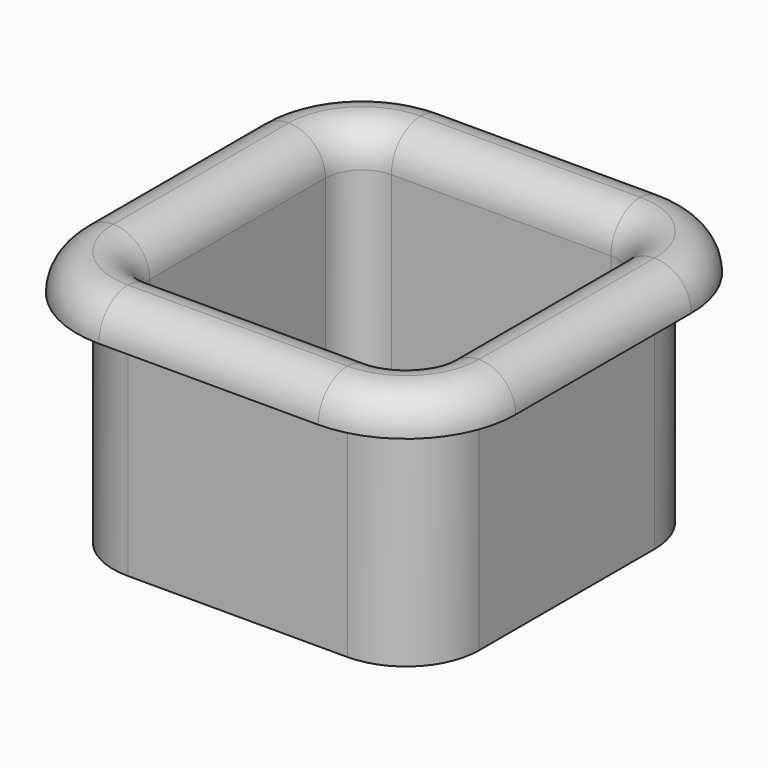
from build123d import *

# Parameters (mm, degrees)
F1_DEPTH = 6.35
F2_DEPTH = 38.1
F3_R     = 6.34999


# Not quite as in the source:
# - a fillet or chamfer is up to 0.001 mm smaller than in the source, because OpenCascade refuses the exact size


with BuildPart() as f1:
    # F0 (on Top) → F1 (new body)
    with BuildSketch(Plane.XY):
        with BuildLine():
            Line((-19.05, -38.1000031829), (19.05, -38.1000031829))
            ThreePointArc((19.05, -38.1000031829), (32.5203864322, -32.5203864322), (38.1000031829, -19.05))
            Line((38.1000031829, -19.05), (38.1000031829, 19.05))
            ThreePointArc((38.1000031829, 19.05), (32.5203864322, 32.5203864322), (19.05, 38.1000031829))
            Line((19.05, 38.1000031829), (-19.05, 38.1000031829))
            ThreePointArc((-19.05, 38.1000031829), (-32.5203864322, 32.5203864322), (-38.1000031829, 19.05))
            Line((-38.1000031829, 19.05), (-38.1000031829, -19.05))
            ThreePointArc((-38.1000031829, -19.05), (-32.5203864322, -32.5203864322), (-19.05, -38.1000031829))
        make_face()
        with BuildLine():
            ThreePointArc((-19.05, -31.75), (-28.0302561211, -28.0302561211), (-31.75, -19.05))
            Line((-31.75, -19.05), (-31.75, 19.05))
            ThreePointArc((-31.75, 19.05), (-28.0302561211, 28.0302561211), (-19.05, 31.75))
            Line((-19.05, 31.75), (19.05, 31.75))
            ThreePointArc((19.05, 31.75), (28.0302561211, 28.0302561211), (31.75, 19.05))
            Line((31.75, 19.05), (31.75, -19.05))
            ThreePointArc((31.75, -19.05), (28.0302561211, -28.0302561211), (19.05, -31.75))
            Line((19.05, -31.75), (-19.05, -31.75))
        make_face(mode=Mode.SUBTRACT)
        with BuildLine():
            Line((-31.75, 19.05), (-31.75, -19.05))
            ThreePointArc((-31.75, -19.05), (-28.0302561211, -28.0302561211), (-19.05, -31.75))
            Line((-19.05, -31.75), (19.05, -31.75))
            ThreePointArc((19.05, -31.75), (28.0302561211, -28.0302561211), (31.75, -19.05))
            Line((31.75, -19.05), (31.75, 19.05))
            ThreePointArc((31.75, 19.05), (28.0302561211, 28.0302561211), (19.05, 31.75))
            Line((19.05, 31.75), (-19.05, 31.75))
            ThreePointArc((-19.05, 31.75), (-28.0302561211, 28.0302561211), (-31.75, 19.05))
        make_face()
        with BuildLine():
            Line((19.05, -25.4), (-19.05, -25.4))
            ThreePointArc((-19.05, -25.4), (-23.5401280605, -23.5401280605), (-25.4, -19.05))
            Line((-25.4, -19.05), (-25.4, 19.05))
            ThreePointArc((-25.4, 19.05), (-23.5401280605, 23.5401280605), (-19.05, 25.4))
            Line((-19.05, 25.4), (19.05, 25.4))
            ThreePointArc((19.05, 25.4), (23.5401280605, 23.5401280605), (25.4, 19.05))
            Line((25.4, 19.05), (25.4, -19.05))
            ThreePointArc((25.4, -19.05), (23.5401280605, -23.5401280605), (19.05, -25.4))
        make_face(mode=Mode.SUBTRACT)
    extrude(amount=F1_DEPTH)

    # F0 (on Top) → F2 (join)
    with BuildSketch(Plane.XY):
        with BuildLine():
            Line((-31.75, 19.05), (-31.75, -19.05))
            ThreePointArc((-31.75, -19.05), (-28.0302561211, -28.0302561211), (-19.05, -31.75))
            Line((-19.05, -31.75), (19.05, -31.75))
            ThreePointArc((19.05, -31.75), (28.0302561211, -28.0302561211), (31.75, -19.05))
            Line((31.75, -19.05), (31.75, 19.05))
            ThreePointArc((31.75, 19.05), (28.0302561211, 28.0302561211), (19.05, 31.75))
            Line((19.05, 31.75), (-19.05, 31.75))
            ThreePointArc((-19.05, 31.75), (-28.0302561211, 28.0302561211), (-31.75, 19.05))
        make_face()
        with BuildLine():
            Line((19.05, -25.4), (-19.05, -25.4))
            ThreePointArc((-19.05, -25.4), (-23.5401280605, -23.5401280605), (-25.4, -19.05))
            Line((-25.4, -19.05), (-25.4, 19.05))
            ThreePointArc((-25.4, 19.05), (-23.5401280605, 23.5401280605), (-19.05, 25.4))
            Line((-19.05, 25.4), (19.05, 25.4))
            ThreePointArc((19.05, 25.4), (23.5401280605, 23.5401280605), (25.4, 19.05))
            Line((25.4, 19.05), (25.4, -19.05))
            ThreePointArc((25.4, -19.05), (23.5401280605, -23.5401280605), (19.05, -25.4))
        make_face(mode=Mode.SUBTRACT)
    extrude(amount=-F2_DEPTH)

    # F3 (radius 6.35 in the source; OpenCascade refuses exactly that, so slightly less here)
    f3_edges = [f1.edges().sort_by_distance(p)[0] for p in [
        (23.540128, -23.540128, 6.35),
        (0, -25.4, 6.35),
        (-23.540128, -23.540128, 6.35),
        (-25.4, 0, 6.35),
        (-23.540128, 23.540128, 6.35),
        (0, 25.4, 6.35),
        (23.540128, 23.540128, 6.35),
        (25.4, 0, 6.35),
        (0, -38.100003, 6.35),
        (32.520386, -32.520386, 6.35),
        (38.100003, 0, 6.35),
        (32.520386, 32.520386, 6.35),
        (0, 38.100003, 6.35),
        (-32.520386, 32.520386, 6.35),
        (-38.100003, 0, 6.35),
        (-32.520386, -32.520386, 6.35),
    ]]
    fillet(f3_edges, radius=F3_R)


solid = f1.part
